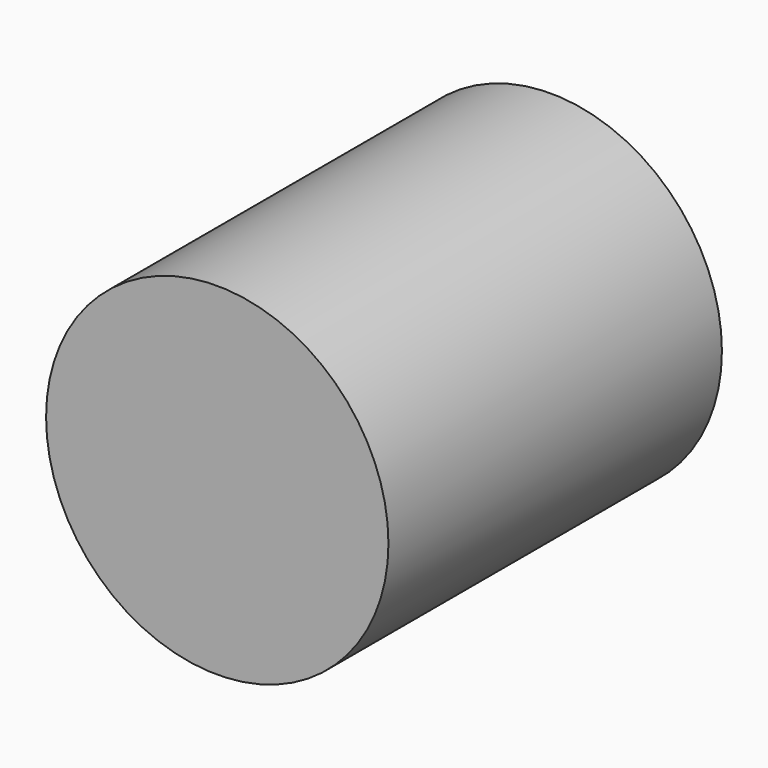
from build123d import *

# Parameters (mm, degrees)
F0_R     = 41.7239859136
F1_DEPTH = 101.6


# Not quite as in the source:
# - the program builds the solid bodies; features that only make, move or delete a surface that nothing else refers to are left out


with BuildPart() as f1:
    # F0 (on Front) → F1 (new body)
    with BuildSketch(Plane.XZ):
        Circle(F0_R)
    extrude(amount=F1_DEPTH)


solid = f1.part
